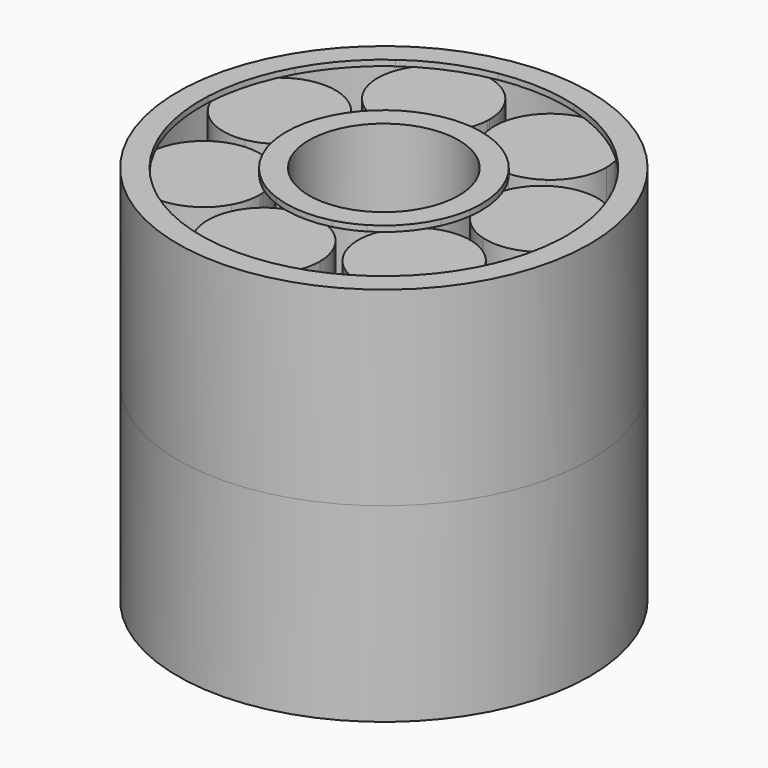
from build123d import *

# Parameters (mm, degrees)
F0_R     = 27.5
F0_R_2   = 26.6334952823
F1_DEPTH = 25.4
F0_R_3   = 10.7610049785
F0_R_4   = 10
F2_DEPTH = 24.638
F3_DEPTH = 24.13


# Not quite as in the source:
# - a feature names something its author has since deleted; it is built from what else it names


with BuildPart() as f1:
    # F0 (on Top) → F1 (new body)
    with BuildSketch(Plane.XY):
        Circle(F0_R)
        Circle(F0_R_2, mode=Mode.SUBTRACT)
        Circle(F0_R_2)
        with BuildLine():
            ThreePointArc((16.3321734228, 18.1725346213), (19.895604505, 14.1825887853), (22.5052921525, 9.5127666008))
            ThreePointArc((22.5052921525, 9.5127666008), (25.0644578024, 6.7999381044), (25.9946749575, 3.1883645805))
            ThreePointArc((25.9946749575, 3.1883645805), (25.5823358734, 0.7398259238), (24.3908032544, -1.4386173488))
            ThreePointArc((24.3908032544, -1.4386173488), (23.4931009259, -6.7123104932), (21.4692005589, -11.6642329639))
            ThreePointArc((21.4692005589, -11.6642329639), (21.5035422894, -12.0767337285), (21.515001242, -12.4905029004))
            ThreePointArc((21.515001242, -12.4905029004), (19.3407501763, -17.7614050131), (14.0826607538, -19.9664611128))
            ThreePointArc((14.0826607538, -19.9664611128), (9.3998131777, -22.5527030641), (4.2663630525, -24.0578271998))
            ThreePointArc((4.2663630525, -24.0578271998), (-1.415114182, -26.2289959572), (-6.8300125284, -23.4591524172))
            ThreePointArc((-6.8300125284, -23.4591524172), (-11.7717256146, -21.4104502364), (-16.1491328504, -18.335386864))
            ThreePointArc((-16.1491328504, -18.335386864), (-21.3889640538, -15.2471306735), (-22.5995470698, -9.286623472))
            ThreePointArc((-22.5995470698, -9.286623472), (-24.0789149197, -4.1456916871), (-24.4040023346, 1.1939737541))
            ThreePointArc((-24.4040023346, 1.1939737541), (-25.2564877377, 7.216134992), (-21.3511617209, 11.8789223602))
            ThreePointArc((-21.3511617209, 11.8789223602), (-18.2541901698, 16.2408572593), (-14.2821603099, 19.8242477828))
            ThreePointArc((-14.2821603099, 19.8242477828), (-10.1053610167, 24.2455038263), (-4.0249161118, 24.0993973693))
            ThreePointArc((-4.0249161118, 24.0993973693), (1.3163120955, 24.3977094363), (6.5944397311, 23.5264588901))
            ThreePointArc((6.5944397311, 23.5264588901), (12.6553086617, 23.0175137612), (16.3321734228, 18.1725346213))
        make_face(mode=Mode.SUBTRACT)
        with BuildLine():
            ThreePointArc((6.5944397311, 23.5264588901), (11.7717256146, 21.4104502364), (16.3321734228, 18.1725346213))
            ThreePointArc((16.3321734228, 18.1725346213), (12.6553086617, 23.0175137612), (6.5944397311, 23.5264588901))
        make_face()
        with BuildLine():
            ThreePointArc((25.9946749575, 3.1883645805), (25.0644578024, 6.7999381044), (22.5052921525, 9.5127666008))
            ThreePointArc((22.5052921525, 9.5127666008), (23.9463675969, 4.85307966), (24.4331926541, 0))
            ThreePointArc((24.4331926541, 0), (24.422593005, -0.7196208615), (24.3908032544, -1.4386173488))
            ThreePointArc((24.3908032544, -1.4386173488), (25.5823358734, 0.7398259238), (25.9946749575, 3.1883645805))
        make_face()
        with BuildLine():
            ThreePointArc((21.515001242, -12.4905029004), (21.5035422894, -12.0767337285), (21.4692005589, -11.6642329639))
            ThreePointArc((21.4692005589, -11.6642329639), (18.2541901698, -16.2408572593), (14.0826607538, -19.9664611128))
            ThreePointArc((14.0826607538, -19.9664611128), (19.3407501763, -17.7614050131), (21.515001242, -12.4905029004))
        make_face()
        with BuildLine():
            ThreePointArc((-6.8300125284, -23.4591524172), (-1.415114182, -26.2289959572), (4.2663630525, -24.0578271998))
            ThreePointArc((4.2663630525, -24.0578271998), (-1.3163120955, -24.3977094363), (-6.8300125284, -23.4591524172))
        make_face()
        with BuildLine():
            ThreePointArc((-22.5995470698, -9.286623472), (-21.3889640538, -15.2471306735), (-16.1491328504, -18.335386864))
            ThreePointArc((-16.1491328504, -18.335386864), (-19.895604505, -14.1825887853), (-22.5995470698, -9.286623472))
        make_face()
        with BuildLine():
            ThreePointArc((-24.4040023346, 1.1939737541), (-23.4931009259, 6.7123104932), (-21.3511617209, 11.8789223602))
            ThreePointArc((-21.3511617209, 11.8789223602), (-25.2564877377, 7.216134992), (-24.4040023346, 1.1939737541))
        make_face()
        with BuildLine():
            ThreePointArc((-14.2821603099, 19.8242477828), (-9.3998131777, 22.5527030641), (-4.0249161118, 24.0993973693))
            ThreePointArc((-4.0249161118, 24.0993973693), (-10.1053610167, 24.2455038263), (-14.2821603099, 19.8242477828))
        make_face()
    extrude(amount=F1_DEPTH)


with BuildPart() as f1b:
    # F0 (on Top) → F1, piece 2 (new body)
    with BuildSketch(Plane.XY):
        with BuildLine():
            ThreePointArc((12.9059413599, -1.7502641846), (11.150904717, 1.9198627988), (11.5774926397, 5.9656023401))
            ThreePointArc((11.5774926397, 5.9656023401), (10.6053275573, 7.5600115413), (9.4151344634, 8.9989993965))
            ThreePointArc((9.4151344634, 8.9989993965), (5.4514661944, 9.9151432418), (2.5543528706, 12.7711404547))
            ThreePointArc((2.5543528706, 12.7711404547), (0.7016585466, 13.0051690641), (-1.1654607178, 12.9718328858))
            ThreePointArc((-1.1654607178, 12.9718328858), (-4.3530375622, 10.4441185916), (-8.3922667094, 9.9597493232))
            ThreePointArc((-8.3922667094, 9.9597493232), (-9.730373661, 8.6571690246), (-10.8684402074, 7.176611635))
            ThreePointArc((-10.8684402074, 7.176611635), (-10.6614065218, 6.1788971039), (-10.5919652925, 5.1622973064))
            ThreePointArc((-10.5919652925, 5.1622973064), (-11.2256659436, 2.150051488), (-13.0193382861, -0.3515361906))
            ThreePointArc((-13.0193382861, -0.3515361906), (-12.8352360383, -2.2098558645), (-12.3872625451, -4.0227445532))
            ThreePointArc((-12.3872625451, -4.0227445532), (-9.2136207492, -6.5679328455), (-7.8425825873, -10.3981077828))
            ThreePointArc((-7.8425825873, -10.3981077828), (-6.2749038878, -11.4128142148), (-4.5782235322, -12.1928920438))
            ThreePointArc((-4.5782235322, -12.1928920438), (-0.609581902, -11.2985379177), (3.2397977593, -12.6146921318))
            ThreePointArc((3.2397977593, -12.6146921318), (5.010558875, -12.0216906823), (6.6783111792, -11.1815431357))
            ThreePointArc((6.6783111792, -11.1815431357), (8.4534845507, -7.5211134897), (11.8825443133, -5.3321560127))
            ThreePointArc((11.8825443133, -5.3321560127), (12.5229686081, -3.5779888683), (12.9059413599, -1.7502641846))
        make_face()
        Circle(F0_R_3, mode=Mode.SUBTRACT)
        Circle(F0_R_3)
        Circle(F0_R_4, mode=Mode.SUBTRACT)
        with BuildLine():
            ThreePointArc((-8.3922667094, 9.9597493232), (-4.3530375622, 10.4441185916), (-1.1654607178, 12.9718328858))
            ThreePointArc((-1.1654607178, 12.9718328858), (-5.010558875, 12.0216906823), (-8.3922667094, 9.9597493232))
        make_face()
        with BuildLine():
            ThreePointArc((2.5543528706, 12.7711404547), (5.4514661944, 9.9151432418), (9.4151344634, 8.9989993965))
            ThreePointArc((9.4151344634, 8.9989993965), (6.2749038878, 11.4128142148), (2.5543528706, 12.7711404547))
        make_face()
        with BuildLine():
            ThreePointArc((12.9059413599, -1.7502641846), (12.9945142864, -0.8771234585), (13.0240833498, 0))
            ThreePointArc((13.0240833498, 0), (12.6572701682, 3.0692440422), (11.5774926397, 5.9656023401))
            ThreePointArc((11.5774926397, 5.9656023401), (11.150904717, 1.9198627988), (12.9059413599, -1.7502641846))
        make_face()
        with BuildLine():
            ThreePointArc((6.6783111792, -11.1815431357), (9.730373661, -8.6571690246), (11.8825443133, -5.3321560127))
            ThreePointArc((11.8825443133, -5.3321560127), (8.4534845507, -7.5211134897), (6.6783111792, -11.1815431357))
        make_face()
        with BuildLine():
            ThreePointArc((-4.5782235322, -12.1928920438), (-0.7016585466, -13.0051690641), (3.2397977593, -12.6146921318))
            ThreePointArc((3.2397977593, -12.6146921318), (-0.609581902, -11.2985379177), (-4.5782235322, -12.1928920438))
        make_face()
        with BuildLine():
            ThreePointArc((-12.3872625451, -4.0227445532), (-10.6053275573, -7.5600115413), (-7.8425825873, -10.3981077828))
            ThreePointArc((-7.8425825873, -10.3981077828), (-9.2136207492, -6.5679328455), (-12.3872625451, -4.0227445532))
        make_face()
        with BuildLine():
            ThreePointArc((-10.5919652925, 5.1622973064), (-10.6614065218, 6.1788971039), (-10.8684402074, 7.176611635))
            ThreePointArc((-10.8684402074, 7.176611635), (-12.5229686081, 3.5779888683), (-13.0193382861, -0.3515361906))
            ThreePointArc((-13.0193382861, -0.3515361906), (-11.2256659436, 2.150051488), (-10.5919652925, 5.1622973064))
        make_face()
    extrude(amount=F1_DEPTH)


with BuildPart() as f2_tool:
    # F0 (on Top) → F2 (new body)
    with BuildSketch(Plane.XY):
        Circle(F0_R_2)
        with BuildLine():
            ThreePointArc((16.3321734228, 18.1725346213), (19.895604505, 14.1825887853), (22.5052921525, 9.5127666008))
            ThreePointArc((22.5052921525, 9.5127666008), (25.0644578024, 6.7999381044), (25.9946749575, 3.1883645805))
            ThreePointArc((25.9946749575, 3.1883645805), (25.5823358734, 0.7398259238), (24.3908032544, -1.4386173488))
            ThreePointArc((24.3908032544, -1.4386173488), (23.4931009259, -6.7123104932), (21.4692005589, -11.6642329639))
            ThreePointArc((21.4692005589, -11.6642329639), (21.5035422894, -12.0767337285), (21.515001242, -12.4905029004))
            ThreePointArc((21.515001242, -12.4905029004), (19.3407501763, -17.7614050131), (14.0826607538, -19.9664611128))
            ThreePointArc((14.0826607538, -19.9664611128), (9.3998131777, -22.5527030641), (4.2663630525, -24.0578271998))
            ThreePointArc((4.2663630525, -24.0578271998), (-1.415114182, -26.2289959572), (-6.8300125284, -23.4591524172))
            ThreePointArc((-6.8300125284, -23.4591524172), (-11.7717256146, -21.4104502364), (-16.1491328504, -18.335386864))
            ThreePointArc((-16.1491328504, -18.335386864), (-21.3889640538, -15.2471306735), (-22.5995470698, -9.286623472))
            ThreePointArc((-22.5995470698, -9.286623472), (-24.0789149197, -4.1456916871), (-24.4040023346, 1.1939737541))
            ThreePointArc((-24.4040023346, 1.1939737541), (-25.2564877377, 7.216134992), (-21.3511617209, 11.8789223602))
            ThreePointArc((-21.3511617209, 11.8789223602), (-18.2541901698, 16.2408572593), (-14.2821603099, 19.8242477828))
            ThreePointArc((-14.2821603099, 19.8242477828), (-10.1053610167, 24.2455038263), (-4.0249161118, 24.0993973693))
            ThreePointArc((-4.0249161118, 24.0993973693), (1.3163120955, 24.3977094363), (6.5944397311, 23.5264588901))
            ThreePointArc((6.5944397311, 23.5264588901), (12.6553086617, 23.0175137612), (16.3321734228, 18.1725346213))
        make_face(mode=Mode.SUBTRACT)
        with BuildLine():
            ThreePointArc((-24.4040023346, 1.1939737541), (-23.4931009259, 6.7123104932), (-21.3511617209, 11.8789223602))
            ThreePointArc((-21.3511617209, 11.8789223602), (-25.2564877377, 7.216134992), (-24.4040023346, 1.1939737541))
        make_face()
        with BuildLine():
            ThreePointArc((-22.5995470698, -9.286623472), (-21.3889640538, -15.2471306735), (-16.1491328504, -18.335386864))
            ThreePointArc((-16.1491328504, -18.335386864), (-19.895604505, -14.1825887853), (-22.5995470698, -9.286623472))
        make_face()
        with BuildLine():
            ThreePointArc((-6.8300125284, -23.4591524172), (-1.415114182, -26.2289959572), (4.2663630525, -24.0578271998))
            ThreePointArc((4.2663630525, -24.0578271998), (-1.3163120955, -24.3977094363), (-6.8300125284, -23.4591524172))
        make_face()
        with BuildLine():
            ThreePointArc((21.515001242, -12.4905029004), (21.5035422894, -12.0767337285), (21.4692005589, -11.6642329639))
            ThreePointArc((21.4692005589, -11.6642329639), (18.2541901698, -16.2408572593), (14.0826607538, -19.9664611128))
            ThreePointArc((14.0826607538, -19.9664611128), (19.3407501763, -17.7614050131), (21.515001242, -12.4905029004))
        make_face()
        with BuildLine():
            ThreePointArc((25.9946749575, 3.1883645805), (25.0644578024, 6.7999381044), (22.5052921525, 9.5127666008))
            ThreePointArc((22.5052921525, 9.5127666008), (23.9463675969, 4.85307966), (24.4331926541, 0))
            ThreePointArc((24.4331926541, 0), (24.422593005, -0.7196208615), (24.3908032544, -1.4386173488))
            ThreePointArc((24.3908032544, -1.4386173488), (25.5823358734, 0.7398259238), (25.9946749575, 3.1883645805))
        make_face()
        with BuildLine():
            ThreePointArc((6.5944397311, 23.5264588901), (11.7717256146, 21.4104502364), (16.3321734228, 18.1725346213))
            ThreePointArc((16.3321734228, 18.1725346213), (12.6553086617, 23.0175137612), (6.5944397311, 23.5264588901))
        make_face()
        with BuildLine():
            ThreePointArc((-14.2821603099, 19.8242477828), (-9.3998131777, 22.5527030641), (-4.0249161118, 24.0993973693))
            ThreePointArc((-4.0249161118, 24.0993973693), (-10.1053610167, 24.2455038263), (-14.2821603099, 19.8242477828))
        make_face()
        with BuildLine():
            ThreePointArc((12.9059413599, -1.7502641846), (11.150904717, 1.9198627988), (11.5774926397, 5.9656023401))
            ThreePointArc((11.5774926397, 5.9656023401), (10.6053275573, 7.5600115413), (9.4151344634, 8.9989993965))
            ThreePointArc((9.4151344634, 8.9989993965), (5.4514661944, 9.9151432418), (2.5543528706, 12.7711404547))
            ThreePointArc((2.5543528706, 12.7711404547), (0.7016585466, 13.0051690641), (-1.1654607178, 12.9718328858))
            ThreePointArc((-1.1654607178, 12.9718328858), (-4.3530375622, 10.4441185916), (-8.3922667094, 9.9597493232))
            ThreePointArc((-8.3922667094, 9.9597493232), (-9.730373661, 8.6571690246), (-10.8684402074, 7.176611635))
            ThreePointArc((-10.8684402074, 7.176611635), (-10.6614065218, 6.1788971039), (-10.5919652925, 5.1622973064))
            ThreePointArc((-10.5919652925, 5.1622973064), (-11.2256659436, 2.150051488), (-13.0193382861, -0.3515361906))
            ThreePointArc((-13.0193382861, -0.3515361906), (-12.8352360383, -2.2098558645), (-12.3872625451, -4.0227445532))
            ThreePointArc((-12.3872625451, -4.0227445532), (-9.2136207492, -6.5679328455), (-7.8425825873, -10.3981077828))
            ThreePointArc((-7.8425825873, -10.3981077828), (-6.2749038878, -11.4128142148), (-4.5782235322, -12.1928920438))
            ThreePointArc((-4.5782235322, -12.1928920438), (-0.609581902, -11.2985379177), (3.2397977593, -12.6146921318))
            ThreePointArc((3.2397977593, -12.6146921318), (5.010558875, -12.0216906823), (6.6783111792, -11.1815431357))
            ThreePointArc((6.6783111792, -11.1815431357), (8.4534845507, -7.5211134897), (11.8825443133, -5.3321560127))
            ThreePointArc((11.8825443133, -5.3321560127), (12.5229686081, -3.5779888683), (12.9059413599, -1.7502641846))
        make_face()
        Circle(F0_R_3, mode=Mode.SUBTRACT)
        with BuildLine():
            ThreePointArc((2.5543528706, 12.7711404547), (5.4514661944, 9.9151432418), (9.4151344634, 8.9989993965))
            ThreePointArc((9.4151344634, 8.9989993965), (6.2749038878, 11.4128142148), (2.5543528706, 12.7711404547))
        make_face()
        with BuildLine():
            ThreePointArc((-8.3922667094, 9.9597493232), (-4.3530375622, 10.4441185916), (-1.1654607178, 12.9718328858))
            ThreePointArc((-1.1654607178, 12.9718328858), (-5.010558875, 12.0216906823), (-8.3922667094, 9.9597493232))
        make_face()
        with BuildLine():
            ThreePointArc((12.9059413599, -1.7502641846), (12.9945142864, -0.8771234585), (13.0240833498, 0))
            ThreePointArc((13.0240833498, 0), (12.6572701682, 3.0692440422), (11.5774926397, 5.9656023401))
            ThreePointArc((11.5774926397, 5.9656023401), (11.150904717, 1.9198627988), (12.9059413599, -1.7502641846))
        make_face()
        with BuildLine():
            ThreePointArc((6.6783111792, -11.1815431357), (9.730373661, -8.6571690246), (11.8825443133, -5.3321560127))
            ThreePointArc((11.8825443133, -5.3321560127), (8.4534845507, -7.5211134897), (6.6783111792, -11.1815431357))
        make_face()
        with BuildLine():
            ThreePointArc((-4.5782235322, -12.1928920438), (-0.7016585466, -13.0051690641), (3.2397977593, -12.6146921318))
            ThreePointArc((3.2397977593, -12.6146921318), (-0.609581902, -11.2985379177), (-4.5782235322, -12.1928920438))
        make_face()
        with BuildLine():
            ThreePointArc((-12.3872625451, -4.0227445532), (-10.6053275573, -7.5600115413), (-7.8425825873, -10.3981077828))
            ThreePointArc((-7.8425825873, -10.3981077828), (-9.2136207492, -6.5679328455), (-12.3872625451, -4.0227445532))
        make_face()
        with BuildLine():
            ThreePointArc((-10.5919652925, 5.1622973064), (-10.6614065218, 6.1788971039), (-10.8684402074, 7.176611635))
            ThreePointArc((-10.8684402074, 7.176611635), (-12.5229686081, 3.5779888683), (-13.0193382861, -0.3515361906))
            ThreePointArc((-13.0193382861, -0.3515361906), (-11.2256659436, 2.150051488), (-10.5919652925, 5.1622973064))
        make_face()
    extrude(amount=F2_DEPTH)


with BuildPart() as f1_1:
    add(f1.part)

    # F2: cut by f2_tool
    add(f2_tool.part, mode=Mode.SUBTRACT)


with BuildPart() as f1b_1:
    add(f1b.part)

    # F2: cut by f2_tool
    add(f2_tool.part, mode=Mode.SUBTRACT)


with BuildPart() as f3:
    # F0 (on Top) → F3 (new body)
    with BuildSketch(Plane.XY):
        with BuildLine():
            ThreePointArc((6.5944397311, 23.5264588901), (11.7717256146, 21.4104502364), (16.3321734228, 18.1725346213))
            ThreePointArc((16.3321734228, 18.1725346213), (12.6553086617, 23.0175137612), (6.5944397311, 23.5264588901))
        make_face()
        with BuildLine():
            Line((9.0533874281, 16.4663285015), (13.3929863421, 10.3786568492))
            ThreePointArc((13.3929863421, 10.3786568492), (15.699253829, 13.0422483825), (16.5294736288, 16.4663285015))
            ThreePointArc((16.5294736288, 16.4663285015), (16.4799847786, 17.325116411), (16.3321734228, 18.1725346213))
            ThreePointArc((16.3321734228, 18.1725346213), (11.7717256146, 21.4104502364), (6.5944397311, 23.5264588901))
            ThreePointArc((6.5944397311, 23.5264588901), (3.0782350818, 20.9595922729), (1.5881584083, 16.8690946415))
            Line((1.5881584083, 16.8690946415), (9.0533874281, 16.4663285015))
        make_face()
        with BuildLine():
            ThreePointArc((2.5543528706, 12.7711404547), (6.2749038878, 11.4128142148), (9.4151344634, 8.9989993965))
            ThreePointArc((9.4151344634, 8.9989993965), (11.5031888702, 9.4030192364), (13.3929863421, 10.3786568492))
            Line((13.3929863421, 10.3786568492), (9.0533874281, 16.4663285015))
            Line((9.0533874281, 16.4663285015), (1.5881584083, 16.8690946415))
            ThreePointArc((1.5881584083, 16.8690946415), (1.7768173952, 14.7506964204), (2.5543528706, 12.7711404547))
        make_face()
        with BuildLine():
            ThreePointArc((2.5543528706, 12.7711404547), (5.4514661944, 9.9151432418), (9.4151344634, 8.9989993965))
            ThreePointArc((9.4151344634, 8.9989993965), (6.2749038878, 11.4128142148), (2.5543528706, 12.7711404547))
        make_face()
    extrude(amount=F3_DEPTH)


with BuildPart() as f3b:
    # F0 (on Top) → F3, piece 2 (new body)
    with BuildSketch(Plane.XY):
        with BuildLine():
            ThreePointArc((-14.2821603099, 19.8242477828), (-9.3998131777, 22.5527030641), (-4.0249161118, 24.0993973693))
            ThreePointArc((-4.0249161118, 24.0993973693), (-10.1053610167, 24.2455038263), (-14.2821603099, 19.8242477828))
        make_face()
        with BuildLine():
            Line((-7.2291992894, 17.344811209), (0.2360297303, 16.942045069))
            ThreePointArc((0.2360297303, 16.942045069), (0.2441721231, 17.1433549843), (0.2468869113, 17.344811209))
            ThreePointArc((0.2468869113, 17.344811209), (-0.9106803915, 21.340832207), (-4.0249161118, 24.0993973693))
            ThreePointArc((-4.0249161118, 24.0993973693), (-9.3998131777, 22.5527030641), (-14.2821603099, 19.8242477828))
            ThreePointArc((-14.2821603099, 19.8242477828), (-14.4676209174, 15.4747531307), (-12.1985887001, 11.7593807183))
            Line((-12.1985887001, 11.7593807183), (-7.2291992894, 17.344811209))
        make_face()
        with BuildLine():
            ThreePointArc((-8.3922667094, 9.9597493232), (-5.010558875, 12.0216906823), (-1.1654607178, 12.9718328858))
            ThreePointArc((-1.1654607178, 12.9718328858), (-0.1794555198, 14.856241808), (0.2360297303, 16.942045069))
            Line((0.2360297303, 16.942045069), (-7.2291992894, 17.344811209))
            Line((-7.2291992894, 17.344811209), (-12.1985887001, 11.7593807183))
            ThreePointArc((-12.1985887001, 11.7593807183), (-10.4247313241, 10.5860805666), (-8.3922667094, 9.9597493232))
        make_face()
        with BuildLine():
            ThreePointArc((-8.3922667094, 9.9597493232), (-4.3530375622, 10.4441185916), (-1.1654607178, 12.9718328858))
            ThreePointArc((-1.1654607178, 12.9718328858), (-5.010558875, 12.0216906823), (-8.3922667094, 9.9597493232))
        make_face()
    extrude(amount=F3_DEPTH)


with BuildPart() as f3c:
    # F0 (on Top) → F3, piece 3 (new body)
    with BuildSketch(Plane.XY):
        with BuildLine():
            Line((-18.0680514932, 5.1622973064), (-13.0986620826, 10.7477277971))
            ThreePointArc((-13.0986620826, 10.7477277971), (-17.0527758382, 12.5691239025), (-21.3511617209, 11.8789223602))
            ThreePointArc((-21.3511617209, 11.8789223602), (-23.4931009259, 6.7123104932), (-24.4040023346, 1.1939737541))
            ThreePointArc((-24.4040023346, 1.1939737541), (-21.1190632802, -1.6628907464), (-16.7995497115, -2.2053867334))
            Line((-16.7995497115, -2.2053867334), (-18.0680514932, 5.1622973064))
        make_face()
        with BuildLine():
            ThreePointArc((-24.4040023346, 1.1939737541), (-23.4931009259, 6.7123104932), (-21.3511617209, 11.8789223602))
            ThreePointArc((-21.3511617209, 11.8789223602), (-25.2564877377, 7.216134992), (-24.4040023346, 1.1939737541))
        make_face()
        with BuildLine():
            ThreePointArc((-13.0193382861, -0.3515361906), (-12.5229686081, 3.5779888683), (-10.8684402074, 7.176611635))
            ThreePointArc((-10.8684402074, 7.176611635), (-11.7269662432, 9.1224112861), (-13.0986620826, 10.7477277971))
            Line((-13.0986620826, 10.7477277971), (-18.0680514932, 5.1622973064))
            Line((-18.0680514932, 5.1622973064), (-16.7995497115, -2.2053867334))
            ThreePointArc((-16.7995497115, -2.2053867334), (-14.7762447306, -1.5500698705), (-13.0193382861, -0.3515361906))
        make_face()
        with BuildLine():
            ThreePointArc((-10.5919652925, 5.1622973064), (-10.6614065218, 6.1788971039), (-10.8684402074, 7.176611635))
            ThreePointArc((-10.8684402074, 7.176611635), (-12.5229686081, 3.5779888683), (-13.0193382861, -0.3515361906))
            ThreePointArc((-13.0193382861, -0.3515361906), (-11.2256659436, 2.150051488), (-10.5919652925, 5.1622973064))
        make_face()
    extrude(amount=F3_DEPTH)


with BuildPart() as f3d:
    # F0 (on Top) → F3, piece 4 (new body)
    with BuildSketch(Plane.XY):
        with BuildLine():
            ThreePointArc((-7.8252062008, -10.9075317595), (-7.8295515603, -10.6526716377), (-7.8425825873, -10.3981077828))
            ThreePointArc((-7.8425825873, -10.3981077828), (-10.6053275573, -7.5600115413), (-12.3872625451, -4.0227445532))
            ThreePointArc((-12.3872625451, -4.0227445532), (-14.4438321989, -3.4807809975), (-16.5697941832, -3.5398477197))
            Line((-16.5697941832, -3.5398477197), (-15.3012924015, -10.9075317595))
            Line((-15.3012924015, -10.9075317595), (-8.7501071418, -14.5094529931))
            ThreePointArc((-8.7501071418, -14.5094529931), (-8.0601222406, -12.7669186426), (-7.8252062008, -10.9075317595))
        make_face()
        with BuildLine():
            ThreePointArc((-12.3872625451, -4.0227445532), (-10.6053275573, -7.5600115413), (-7.8425825873, -10.3981077828))
            ThreePointArc((-7.8425825873, -10.3981077828), (-9.2136207492, -6.5679328455), (-12.3872625451, -4.0227445532))
        make_face()
        with BuildLine():
            ThreePointArc((-16.1491328504, -18.335386864), (-11.8674202426, -17.5483439746), (-8.7501071418, -14.5094529931))
            Line((-8.7501071418, -14.5094529931), (-15.3012924015, -10.9075317595))
            Line((-15.3012924015, -10.9075317595), (-16.5697941832, -3.5398477197))
            ThreePointArc((-16.5697941832, -3.5398477197), (-20.4591686026, -5.4956764423), (-22.5995470698, -9.286623472))
            ThreePointArc((-22.5995470698, -9.286623472), (-19.895604505, -14.1825887853), (-16.1491328504, -18.335386864))
        make_face()
        with BuildLine():
            ThreePointArc((-22.5995470698, -9.286623472), (-21.3889640538, -15.2471306735), (-16.1491328504, -18.335386864))
            ThreePointArc((-16.1491328504, -18.335386864), (-19.895604505, -14.1825887853), (-22.5995470698, -9.286623472))
        make_face()
    extrude(amount=F3_DEPTH)


with BuildPart() as f3e:
    # F0 (on Top) → F3, piece 5 (new body)
    with BuildSketch(Plane.XY):
        with BuildLine():
            ThreePointArc((11.5774926397, 5.9656023401), (12.6572701682, 3.0692440422), (13.0240833498, 0))
            ThreePointArc((13.0240833498, 0), (12.9945142864, -0.8771234585), (12.9059413599, -1.7502641846))
            ThreePointArc((12.9059413599, -1.7502641846), (14.5236974186, -3.1308686069), (16.4647510712, -4.000071664))
            Line((16.4647510712, -4.000071664), (18.5185887568, 3.1883645805))
            Line((18.5185887568, 3.1883645805), (14.1789898428, 9.2760362328))
            ThreePointArc((14.1789898428, 9.2760362328), (12.6403863755, 7.8077370102), (11.5774926397, 5.9656023401))
        make_face()
        with BuildLine():
            ThreePointArc((22.5052921525, 9.5127666008), (18.3061172799, 10.6614309359), (14.1789898428, 9.2760362328))
            Line((14.1789898428, 9.2760362328), (18.5185887568, 3.1883645805))
            Line((18.5185887568, 3.1883645805), (16.4647510712, -4.000071664))
            ThreePointArc((16.4647510712, -4.000071664), (20.8175586178, -3.92546719), (24.3908032544, -1.4386173488))
            ThreePointArc((24.3908032544, -1.4386173488), (24.422593005, -0.7196208615), (24.4331926541, 0))
            ThreePointArc((24.4331926541, 0), (23.9463675969, 4.85307966), (22.5052921525, 9.5127666008))
        make_face()
        with BuildLine():
            ThreePointArc((25.9946749575, 3.1883645805), (25.0644578024, 6.7999381044), (22.5052921525, 9.5127666008))
            ThreePointArc((22.5052921525, 9.5127666008), (23.9463675969, 4.85307966), (24.4331926541, 0))
            ThreePointArc((24.4331926541, 0), (24.422593005, -0.7196208615), (24.3908032544, -1.4386173488))
            ThreePointArc((24.3908032544, -1.4386173488), (25.5823358734, 0.7398259238), (25.9946749575, 3.1883645805))
        make_face()
        with BuildLine():
            ThreePointArc((12.9059413599, -1.7502641846), (12.9945142864, -0.8771234585), (13.0240833498, 0))
            ThreePointArc((13.0240833498, 0), (12.6572701682, 3.0692440422), (11.5774926397, 5.9656023401))
            ThreePointArc((11.5774926397, 5.9656023401), (11.150904717, 1.9198627988), (12.9059413599, -1.7502641846))
        make_face()
    extrude(amount=F3_DEPTH)


with BuildPart() as f3f:
    # F0 (on Top) → F3, piece 6 (new body)
    with BuildSketch(Plane.XY):
        with BuildLine():
            ThreePointArc((6.6783111792, -11.1815431357), (9.730373661, -8.6571690246), (11.8825443133, -5.3321560127))
            ThreePointArc((11.8825443133, -5.3321560127), (8.4534845507, -7.5211134897), (6.6783111792, -11.1815431357))
        make_face()
        with BuildLine():
            ThreePointArc((16.0927527269, -5.3020666559), (13.9854865981, -5.0146076174), (11.8825443133, -5.3321560127))
            ThreePointArc((11.8825443133, -5.3321560127), (9.730373661, -8.6571690246), (6.6783111792, -11.1815431357))
            ThreePointArc((6.6783111792, -11.1815431357), (6.6075655815, -13.3071485311), (7.138222424, -15.3666646277))
            Line((7.138222424, -15.3666646277), (14.0389150413, -12.4905029004))
            Line((14.0389150413, -12.4905029004), (16.0927527269, -5.3020666559))
        make_face()
        with BuildLine():
            ThreePointArc((21.4692005589, -11.6642329639), (19.7491197895, -7.6650053494), (16.0927527269, -5.3020666559))
            Line((16.0927527269, -5.3020666559), (14.0389150413, -12.4905029004))
            Line((14.0389150413, -12.4905029004), (7.138222424, -15.3666646277))
            ThreePointArc((7.138222424, -15.3666646277), (9.9104816653, -18.723311476), (14.0826607538, -19.9664611128))
            ThreePointArc((14.0826607538, -19.9664611128), (18.2541901698, -16.2408572593), (21.4692005589, -11.6642329639))
        make_face()
        with BuildLine():
            ThreePointArc((21.515001242, -12.4905029004), (21.5035422894, -12.0767337285), (21.4692005589, -11.6642329639))
            ThreePointArc((21.4692005589, -11.6642329639), (18.2541901698, -16.2408572593), (14.0826607538, -19.9664611128))
            ThreePointArc((14.0826607538, -19.9664611128), (19.3407501763, -17.7614050131), (21.515001242, -12.4905029004))
        make_face()
    extrude(amount=F3_DEPTH)


with BuildPart() as f3g:
    # F0 (on Top) → F3, piece 7 (new body)
    with BuildSketch(Plane.XY):
        with BuildLine():
            ThreePointArc((-4.5782235322, -12.1928920438), (-0.7016585466, -13.0051690641), (3.2397977593, -12.6146921318))
            ThreePointArc((3.2397977593, -12.6146921318), (-0.609581902, -11.2985379177), (-4.5782235322, -12.1928920438))
        make_face()
        with BuildLine():
            ThreePointArc((5.8883445754, -15.8876052102), (4.7992301604, -14.0608504298), (3.2397977593, -12.6146921318))
            ThreePointArc((3.2397977593, -12.6146921318), (-0.7016585466, -13.0051690641), (-4.5782235322, -12.1928920438))
            ThreePointArc((-4.5782235322, -12.1928920438), (-6.2841979083, -13.462874195), (-7.5635333017, -15.1618457038))
            Line((-7.5635333017, -15.1618457038), (-1.012348042, -18.7637669375))
            Line((-1.012348042, -18.7637669375), (5.8883445754, -15.8876052102))
        make_face()
        with BuildLine():
            ThreePointArc((6.4637381587, -18.7637669375), (6.3184785735, -17.2971906475), (5.8883445754, -15.8876052102))
            Line((5.8883445754, -15.8876052102), (-1.012348042, -18.7637669375))
            Line((-1.012348042, -18.7637669375), (-7.5635333017, -15.1618457038))
            ThreePointArc((-7.5635333017, -15.1618457038), (-8.4593901182, -19.4221203347), (-6.8300125284, -23.4591524172))
            ThreePointArc((-6.8300125284, -23.4591524172), (-1.3163120955, -24.3977094363), (4.2663630525, -24.0578271998))
            ThreePointArc((4.2663630525, -24.0578271998), (5.8925764345, -21.6297541766), (6.4637381587, -18.7637669375))
        make_face()
        with BuildLine():
            ThreePointArc((-6.8300125284, -23.4591524172), (-1.415114182, -26.2289959572), (4.2663630525, -24.0578271998))
            ThreePointArc((4.2663630525, -24.0578271998), (-1.3163120955, -24.3977094363), (-6.8300125284, -23.4591524172))
        make_face()
    extrude(amount=F3_DEPTH)


with BuildPart() as f4_1:
    # F4: instance of F3d
    add(f3d.part.mirror(Plane.XY))


with BuildPart() as f4_2:
    # F4: instance of F3c
    add(f3c.part.mirror(Plane.XY))


with BuildPart() as f4_3:
    # F4: instance of F3b
    add(f3b.part.mirror(Plane.XY))


with BuildPart() as f4_4:
    # F4: instance of F3g
    add(f3g.part.mirror(Plane.XY))


with BuildPart() as f4_5:
    # F4: instance of F3f
    add(f3f.part.mirror(Plane.XY))


with BuildPart() as f4_6:
    # F4: instance of F3
    add(f3.part.mirror(Plane.XY))


with BuildPart() as f4_7:
    # F4: instance of F3e
    add(f3e.part.mirror(Plane.XY))


with BuildPart() as f4_8:
    # F4: instance of F1
    add(f1_1.part.mirror(Plane.XY))


with BuildPart() as f4_9:
    # F4: instance of F1b
    add(f1b_1.part.mirror(Plane.XY))


solid = Compound([f1_1.part, f1b_1.part, f3.part, f3b.part, f3c.part, f3d.part, f3e.part, f3f.part, f3g.part, f4_1.part, f4_2.part, f4_3.part, f4_4.part, f4_5.part, f4_6.part, f4_7.part, f4_8.part, f4_9.part])
